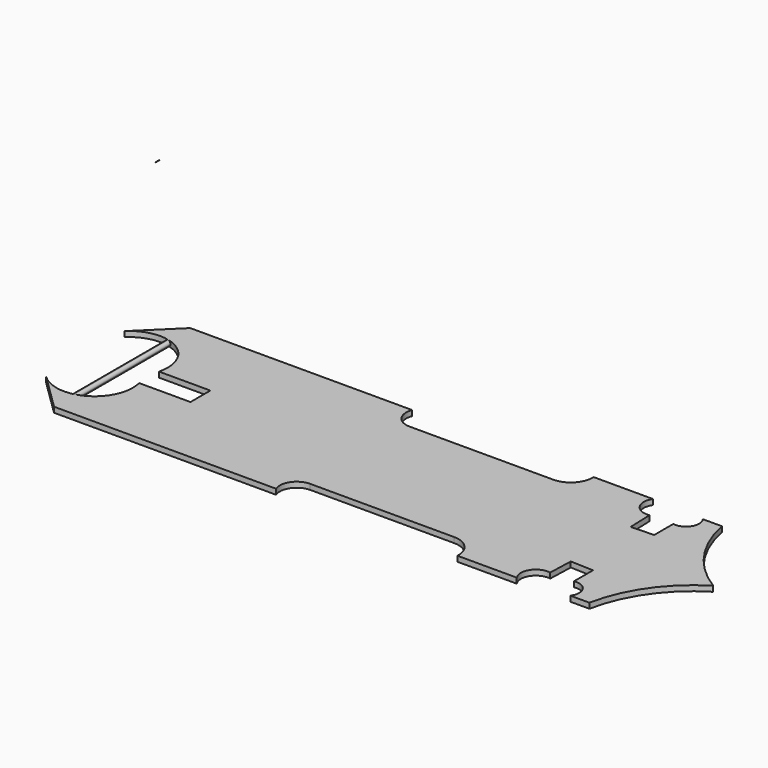
from build123d import *

# Parameters (mm, degrees)
F1_DEPTH = 12.7
F3_DEPTH = 25.4
F4_ANGLE = -90
F6_DEPTH = 12.7
F7_R     = 6.34999
F9_DEPTH = 25.4


# Not quite as in the source:
# - a fillet or chamfer is up to 0.001 mm smaller than in the source, because OpenCascade refuses the exact size


with BuildPart() as f1:
    # F0 (on Front) → F1 (new body)
    with BuildSketch(Plane.XZ):
        with BuildLine():
            ThreePointArc((-551.5071092971, 133.0818972722), (-553.4774467821, 131.195514327), (-555.3919033624, 129.2524429377))
            Line((-555.3919033624, 129.2524429377), (-551.5071092971, 133.0818972722))
        make_face()
    extrude(amount=F1_DEPTH)


with BuildPart() as f1b:
    # F0 (on Front) → F1, piece 2 (new body)
    with BuildSketch(Plane.XZ):
        with BuildLine():
            Line((-453.7474366549, 229.4489622575), (-551.5071092971, 133.0818972722))
            ThreePointArc((-551.5071092971, 133.0818972722), (-421.2871550244, 130.2472203685), (-420.3209924027, 0))
            ThreePointArc((-420.3209924027, 0), (-437.2739000343, -120.3876548814), (-558.7522743609, -115.5303823993))
            Line((-558.7522743609, -115.5303823993), (-471.4288946656, -201.1237346153))
            Line((-471.4288946656, -201.1237346153), (55.251994791, -201.1237346153))
            ThreePointArc((55.251994791, -201.1237346153), (59.5020266904, -163.8701869369), (92.6602373357, -146.3652547012))
            Line((92.6602373357, -146.3652547012), (433.9113681994, -146.3652547012))
            ThreePointArc((433.9113681994, -146.3652547012), (471.5831439124, -162.596085617), (485.6623065385, -201.1237346153))
            Line((485.6623065385, -201.1237346153), (626.4786631969, -201.1237346153))
            ThreePointArc((626.4786631969, -201.1237346153), (626.2028327697, -161.9974569275), (662.0717042558, -146.3652547012))
            Line((662.0717042558, -146.3652547012), (664.0649618373, -87.9562156213))
            Line((664.0649618373, -87.9562156213), (718.4053118981, -89.8106257683))
            Line((718.4053118981, -89.8106257683), (718.4053118981, -146.3652547012))
            ThreePointArc((718.4053118981, -146.3652547012), (750.4967470004, -160.5430728915), (749.1668792481, -195.6016265885))
            Line((749.1668792481, -195.6016265885), (794.5158585675, -195.6016265885))
            ThreePointArc((794.5158585675, -195.6016265885), (855.3282500186, -65.2281359399), (970.4922497392, 20.9846658139))
            Line((970.4922497392, 20.9846658139), (1027.914232903, 45.041990274))
            Line((1027.914232903, 45.041990274), (970.3385240831, 64.0667292165))
            ThreePointArc((970.3385240831, 64.0667292165), (860.0446545539, 126.9892643459), (785.0380322682, 229.4489622575))
            Line((785.0380322682, 229.4489622575), (736.1340486713, 229.4489622575))
            ThreePointArc((736.1340486713, 229.4489622575), (741.0762182682, 198.5184113591), (715.5427964992, 180.3754129308))
            Line((715.5427964992, 180.3754129308), (715.5427964992, 124.8339117276))
            Line((715.5427964992, 124.8339117276), (664.0649618373, 124.8339117276))
            Line((664.0649618373, 124.8339117276), (664.0649618373, 180.3754129308))
            ThreePointArc((664.0649618373, 180.3754129308), (638.4145031933, 198.2409293595), (640.1981479333, 229.4489622575))
            Line((640.1981479333, 229.4489622575), (469.6364638671, 229.4489622575))
            ThreePointArc((469.6364638671, 229.4489622575), (456.2733947157, 194.8460388869), (422.1188209756, 180.3754129308))
            Line((422.1188209756, 180.3754129308), (92.6602373357, 180.3754129308))
            ThreePointArc((92.6602373357, 180.3754129308), (61.501921171, 195.5559509867), (54.2525633451, 229.4489622575))
            Line((54.2525633451, 229.4489622575), (-453.7474366549, 229.4489622575))
        make_face()
    extrude(amount=F1_DEPTH)

    # F2 (on face) → F3 (cut)
    with BuildSketch(Plane.XZ.offset(12.7)):
        with BuildLine():
            Line((-285.7219224498, 30.356762849), (-400.8898424865, 30.356762849))
            ThreePointArc((-400.8898424865, 30.356762849), (-409.1284035376, 14.232955234), (-420.3209924027, 0))
            ThreePointArc((-420.3209924027, 0), (-412.6608440211, -13.7391565158), (-407.4924357678, -28.5961363948))
            Line((-407.4924357678, -28.5961363948), (-285.7219224498, -28.5961363948))
            Line((-285.7219224498, -28.5961363948), (-285.7219224498, 30.356762849))
        make_face()
    extrude(amount=-F3_DEPTH, mode=Mode.SUBTRACT)


with BuildPart() as f1b_1:
    # F4: moved
    add(f1b.part.rotate(Axis((-208.0884499373, -12.7, -201.1237346153), (-1, 0, 0)), F4_ANGLE))

    # F5 (on face) → F6 (join)
    with BuildSketch(Plane.XY.offset(-188.4237346153)):
        with BuildLine():
            ThreePointArc((-467.190702687, -76.8733791477), (-473.483667963, -75.0662676156), (-479.890702687, -73.7183172825))
            Line((-479.890702687, -73.7183172825), (-479.890702687, -222.6516499079))
            Line((-479.890702687, -222.6516499079), (-467.190702687, -222.6516499079))
            Line((-467.190702687, -222.6516499079), (-467.190702687, -76.8733791477))
        make_face()
    extrude(amount=-F6_DEPTH)

    # F7 (radius 6.35 in the source; OpenCascade refuses exactly that, so slightly less here)
    f7_edges = [f1b_1.edges().sort_by_distance(p)[0] for p in [
        (-467.190703, -149.762515, -201.123735),
        (-467.190703, -149.762515, -188.423735),
        (-479.890703, -148.184984, -188.423735),
        (-479.890703, -148.184984, -201.123735),
    ]]
    fillet(f7_edges, radius=F7_R)

    # F8 (on face) → F9 (cut)
    with BuildSketch(Plane.XY.offset(-188.4237346153)):
        with BuildLine():
            Line((931.0774667122, -214.7040478424), (-285.7219224498, -214.7040478424))
            Line((-285.7219224498, -214.7040478424), (-285.7219224498, -244.1804974643))
            Line((-285.7219224498, -244.1804974643), (-400.8898424865, -244.1804974643))
            ThreePointArc((-400.8898424865, -244.1804974643), (-435.1874662946, -355.6740755463), (-551.5071092971, -346.9056318875))
            Line((-551.5071092971, -346.9056318875), (-453.7474366549, -443.2726968728))
            Line((-453.7474366549, -443.2726968728), (54.2525633451, -443.2726968728))
            ThreePointArc((54.2525633451, -443.2726968728), (61.501921171, -409.379685602), (92.6602373357, -394.1991475461))
            Line((92.6602373357, -394.1991475461), (422.1188209756, -394.1991475461))
            ThreePointArc((422.1188209756, -394.1991475461), (456.2733947157, -408.6697735022), (469.6364638671, -443.2726968728))
            Line((469.6364638671, -443.2726968728), (640.1981479333, -443.2726968728))
            ThreePointArc((640.1981479333, -443.2726968728), (638.4145031933, -412.0646639748), (664.0649618373, -394.1991475461))
            Line((664.0649618373, -394.1991475461), (664.0649618373, -338.6576463429))
            Line((664.0649618373, -338.6576463429), (715.5427964992, -338.6576463429))
            Line((715.5427964992, -338.6576463429), (715.5427964992, -394.1991475461))
            ThreePointArc((715.5427964992, -394.1991475461), (741.0762182682, -412.3421459744), (736.1340486713, -443.2726968728))
            Line((736.1340486713, -443.2726968728), (785.0380322682, -443.2726968728))
            ThreePointArc((785.0380322682, -443.2726968728), (860.0446545539, -340.8129989612), (970.3385240831, -277.8904638318))
            Line((970.3385240831, -277.8904638318), (1027.914232903, -258.8657248893))
            Line((1027.914232903, -258.8657248893), (970.4922497392, -234.8084004292))
            ThreePointArc((970.4922497392, -234.8084004292), (950.408070054, -225.4949210906), (931.0774667122, -214.7040478424))
        make_face()
    extrude(amount=-F9_DEPTH, mode=Mode.SUBTRACT)

    # F10: F1b across face


with BuildPart() as f1b_2:
    add(f1b_1.part)
    add(f1b_1.part.mirror(Plane(origin=(322.6777721312, -214.7040478424, -194.7737346153), x_dir=(1, 0, 0), z_dir=(0, -1, 0))))


solid = Compound([f1.part, f1b_2.part])
